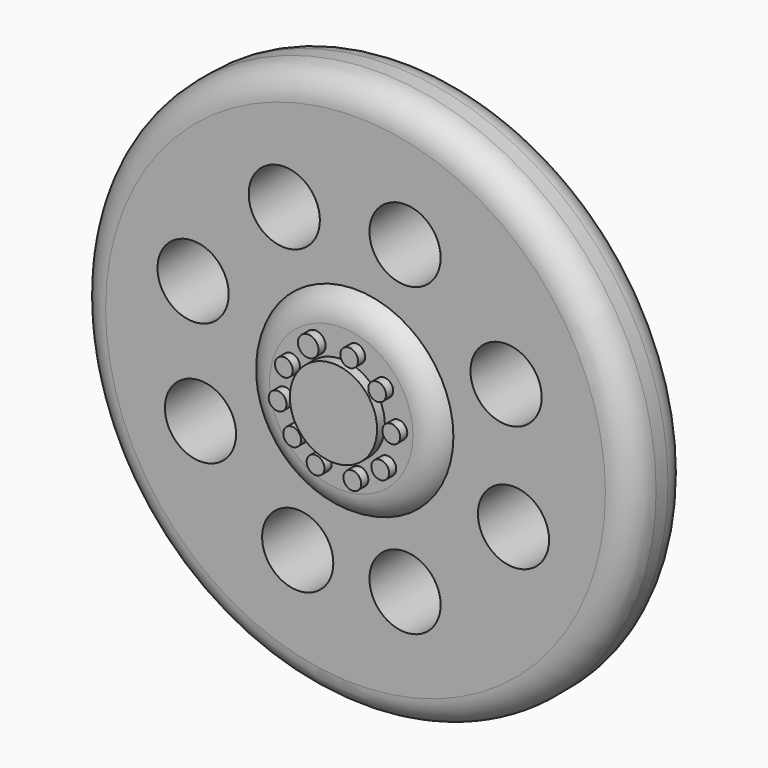
from build123d import *

# Parameters (mm, degrees)
F0_R      = 15.625
F1_DEPTH  = 4
F2_R      = 2.4511
F3_DEPTH  = 1.55
F4_R      = 3
F5_DEPTH  = 9.1
F6_R      = 1.171580863
F7_DEPTH  = 6
F8_R      = 5.5
F9_DEPTH  = 1
F11_R     = 0.5
F11_R_2   = 0.5786516817
F12_DEPTH = 0.5
F13_R     = 2
F14_DEPTH = 25.4


# Not quite as in the source:
# - a fillet or chamfer that OpenCascade refuses, or shapes differently, is made with other operations: its cross-section is extruded or revolved along the edge and cut away or added


with BuildPart() as f1:
    # F0 (on Front) → F1 (new body)
    with BuildSketch(Plane.XZ):
        Circle(F0_R)
    extrude(amount=F1_DEPTH)

    # F2 (on face) → F3 (join)
    with BuildSketch(Plane.XZ.offset(4)):
        Circle(F2_R)
    extrude(amount=F3_DEPTH)

    # F4 (on face) → F5 (join)
    with BuildSketch(Plane(origin=(0, 0, 0), x_dir=(-1, 0, 0), z_dir=(0, 1, 0))):
        Circle(F4_R)
    extrude(amount=F5_DEPTH)

    # F6 (on face) → F7 (cut)
    with BuildSketch(Plane(origin=(0, 9.1, 0), x_dir=(-1, 0, 0), z_dir=(0, 1, 0))):
        Circle(F6_R)
    extrude(amount=-F7_DEPTH, mode=Mode.SUBTRACT)

    # F8 (on face) → F9 (join)
    with BuildSketch(Plane.XZ.offset(4)):
        Circle(F8_R)
    extrude(amount=F9_DEPTH)

    # F10: fillet of radius 1.58242 on 3 edges, made by hand

    # F10_s1 → F10_t2 (revolve, cut)
    with BuildSketch(Plane.XY):
        with BuildLine():
            ThreePointArc((15.625, -2.41758), (15.1615199127, -3.5365199127), (14.04258, -4))
            Line((14.04258, -4), (15.625, -4))
            Line((15.625, -4), (15.625, -2.41758))
        make_face()
    revolve(axis=Axis((0, -4, 0), (0, -1, 0)), mode=Mode.SUBTRACT)

    # F10_s3 → F10_t4 (revolve, cut)
    with BuildSketch(Plane.XY):
        with BuildLine():
            ThreePointArc((15.625, -1.58242), (15.1615199127, -0.4634800873), (14.04258, 0))
            Line((14.04258, 0), (15.625, 0))
            Line((15.625, 0), (15.625, -1.58242))
        make_face()
    revolve(axis=Axis((0, 0, 0), (0, -1, 0)), mode=Mode.SUBTRACT)

    # F10_s5 → F10_t6 (revolve, cut)
    with BuildSketch(Plane.XY):
        with BuildLine():
            ThreePointArc((5.5, -4), (4.9181603337, -4.7263363014), (4.0286604743, -5))
            Line((4.0286604743, -5), (5.5, -5))
            Line((5.5, -5), (5.5, -4))
        make_face()
    revolve(axis=Axis((0, -5, 0), (0, -1, 0)), mode=Mode.SUBTRACT)

    # F11 (on face) → F12 (join)
    with BuildSketch(Plane.XZ.offset(5)):
        with Locations((-2.8265540022, 1.3354053954)):
            Circle(F11_R)
        with Locations((-1.4595896937, 2.8208354488)):
            Circle(F11_R_2)
        with Locations((2.4141243193, 1.8303584075)):
            Circle(F11_R)
        with Locations((3.2077198848, 0)):
            Circle(F11_R)
        with Locations((2.5885446352, -1.9824508684)):
            Circle(F11_R)
        with Locations((1.0188785489, -3.0214018971)):
            Circle(F11_R)
        with Locations((-1.0465403436, -2.928553993)):
            Circle(F11_R)
        with Locations((-3.1790773666, -0.4500864609)):
            Circle(F11_R)
        with Locations((0.8419207879, 2.9949534219)):
            Circle(F11_R)
        with Locations((-2.3607159965, -1.9545760006)):
            Circle(F11_R)
    extrude(amount=F12_DEPTH)

    # F13 (on face) → F14 (cut)
    with BuildSketch(Plane.XZ.offset(4)):
        with Locations((-4.0041380562, 8.2640713081)):
            Circle(F13_R)
        with Locations((2.7820917312, 8.610307239)):
            Circle(F13_R)
        with Locations((-9.1284336522, 2.9320335016)):
            Circle(F13_R)
        with Locations((8.4603661671, 3.555258736)):
            Circle(F13_R)
        with Locations((8.8758496568, -3.3694657031)):
            Circle(F13_R)
        with Locations((2.7820917312, -8.5630090907)):
            Circle(F13_R)
        with Locations((-3.2498515921, -8.4628218188)):
            Circle(F13_R)
        with Locations((-8.7129501626, -3.8541962858)):
            Circle(F13_R)
    extrude(amount=-F14_DEPTH, mode=Mode.SUBTRACT)


solid = f1.part
